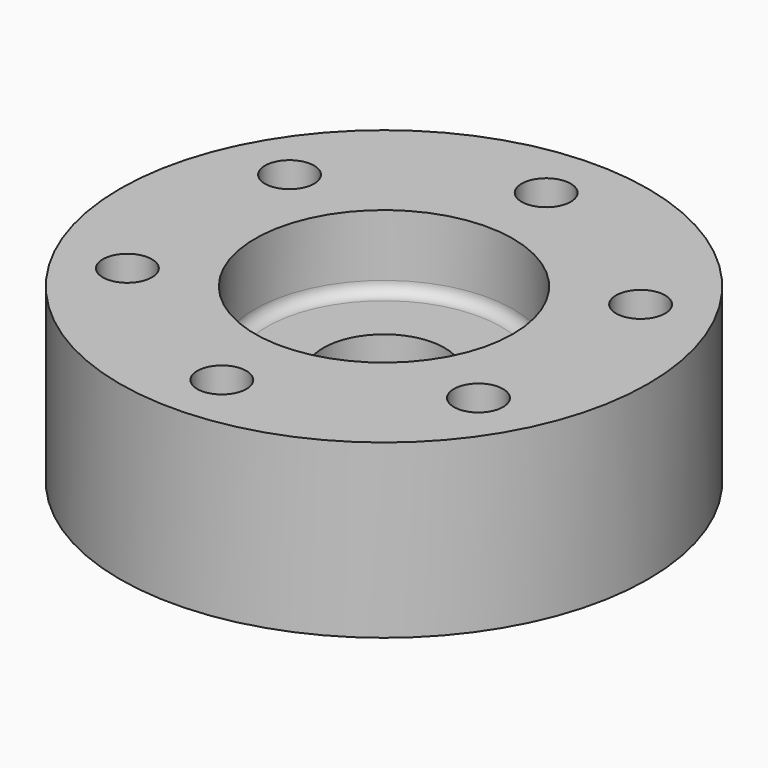
from build123d import *

# Parameters (mm, degrees)
F2_R            = 3.175
F3_DEPTH        = 22.226
F3_COPIES_COUNT = 6


# Not quite as in the source:
# - a pattern or mirror of a feature is missing from the dataset's text; its kind, count and spacing are read off the source's solid


with BuildPart() as f1:
    # F0 (on Front) → F1 (revolve)
    with BuildSketch(Plane.XZ):
        with BuildLine():
            Line((7.8105, 0), (34.1376, 0))
            Line((34.1376, 0), (34.1376, 22.225))
            Line((34.1376, 22.225), (16.6751, 22.225))
            Line((16.6751, 22.225), (16.6751, 14.224))
            ThreePointArc((16.6751, 14.224), (16.2287307345, 13.1463692655), (15.1511, 12.7))
            Line((15.1511, 12.7), (7.8105, 12.7))
            Line((7.8105, 12.7), (7.8105, 0))
        make_face()
    revolve(axis=Axis((0, 0, 6.35), (0, 0, 1)))

    # F2 (on face) → F3 (cut, through all)
    with BuildSketch(Plane.XY.offset(22.225)):
        with Locations((0, 26.2001)):
            Circle(F2_R)
    f3 = extrude(amount=-F3_DEPTH, mode=Mode.SUBTRACT)

    # F3_copies: F3 ×6 about axis
    f3_copies_axis = Axis((0, 0, 0), (0, 0, 1))
    for i in range(1, F3_COPIES_COUNT):
        add(f3.rotate(f3_copies_axis, i * 360 / F3_COPIES_COUNT), mode=Mode.SUBTRACT)


solid = f1.part
